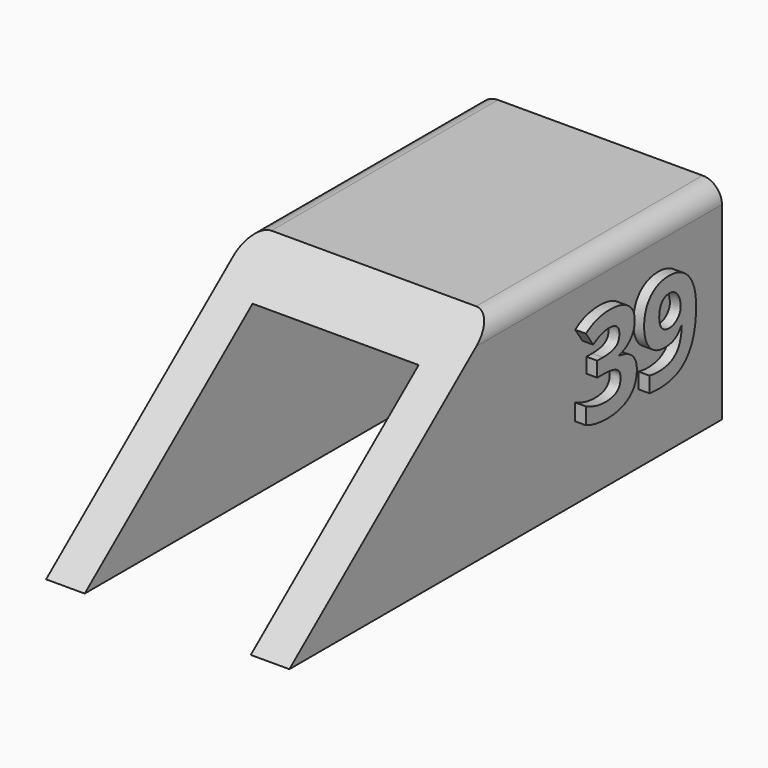
from build123d import *

# Parameters (mm, degrees)
F1_DEPTH      = 50.8
F1_DEPTH_BACK = 38.1
F3_DEPTH      = 40.006
F4_TEXT_SIZE  = 21.2022659576
F5_DEPTH      = 1.778
F6_R          = 3.175


# Not quite as in the source:
# - Text() gives the source's letters only with a copy of the font that has no kerning and outlines rounded to 1/6400 em; it was checked with that copy


with BuildPart() as f1:
    # F0 (on Front) → F1 (new body, two sides)
    with BuildSketch(Plane.XZ) as f1_sk:
        Polygon((0, 34.29), (0, 0), (6.35, 0), (6.35, 27.94), (33.655, 27.94), (33.655, 0), (40.005, 0), (40.005, 34.29), align=None)
    extrude(amount=F1_DEPTH)
    extrude(f1_sk.sketch, amount=-F1_DEPTH_BACK)

    # F2 (on face) → F3 (cut, through all)
    with BuildSketch(Plane.YZ.offset(40.005)):
        Polygon((-50.8, 0), (-8.4553765024, 34.29), (-50.8, 34.29), align=None)
    extrude(amount=-F3_DEPTH, mode=Mode.SUBTRACT)

    # F4 (on face) → F5 (join)
    with BuildSketch(Plane.YZ.offset(40.005)):
        with Locations((7.1084685624, 11.409255676)):
            Text('39', F4_TEXT_SIZE, font='Open Sans', font_style=FontStyle.BOLD, text_align=(TextAlign.LEFT, TextAlign.BOTTOM))
    extrude(amount=F5_DEPTH)

    # F6
    f6_edges = [f1.edges().sort_by_distance(p)[0] for p in [
        (40.005, 14.822312, 34.29),
        (0, 14.822312, 34.29),
    ]]
    fillet(f6_edges, radius=F6_R)


solid = f1.part
